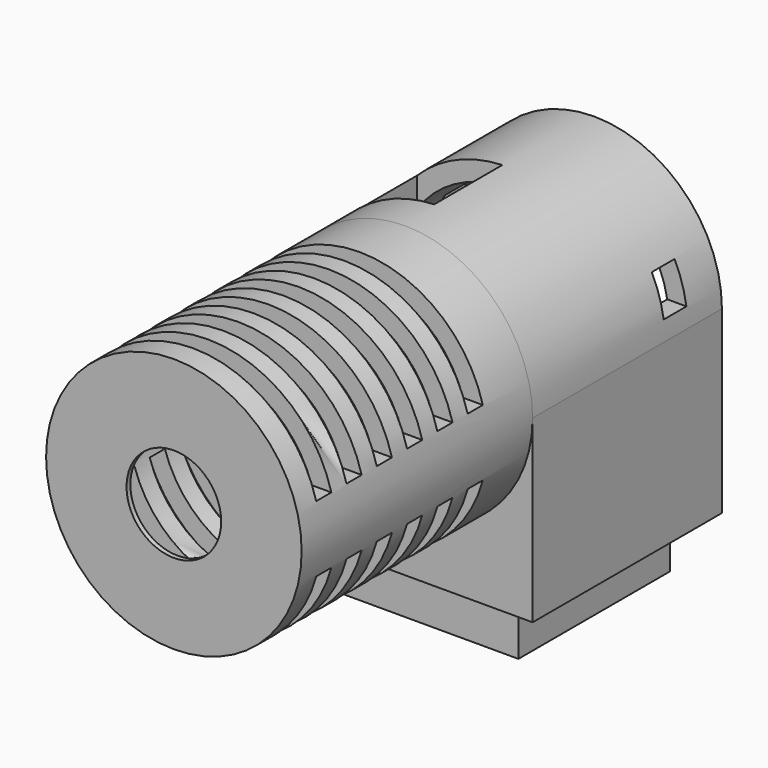
from build123d import *
from build123d import SkipClean  # not in build123d's __all__

# Parameters (mm, degrees)
F0_R      = 13.5
F0_R_2    = 11.5
F1_DEPTH  = 30
F2_R      = 13.5
F2_R_2    = 5
F3_DEPTH  = 0.5
F5_W      = 27
F5_H      = 2
F6_DEPTH  = 10
F8_W      = 27
F8_H      = 2
F9_DEPTH  = 10
F11_DEPTH = 25
F13_DEPTH = 1
F14_W     = 20
F14_H     = 20
F15_DEPTH = 5.55625
F16_W     = 3
F16_H     = 4
F17_DEPTH = 4
F18_W     = 3
F18_H     = 4
F19_DEPTH = 4
F20_W     = 9
F20_H     = 9
F21_DEPTH = 8


# Not quite as in the source:
# - after a boolean that leaves OpenCascade's solid faulty, fix() repairs it
# - a length typed as a fraction of an inch, garbled in the dataset ("3 / 203.2 mm" for 3/8 in), is restored


with BuildPart() as f1:
    # F0 (on Front) → F1 (new body)
    with BuildSketch(Plane.XZ):
        Circle(F0_R)
        Circle(F0_R_2, mode=Mode.SUBTRACT)
    extrude(amount=-F1_DEPTH)

    # F2 (on Front) → F3 (join)
    with BuildSketch(Plane.XZ):
        Circle(F2_R)
        Circle(F2_R_2, mode=Mode.SUBTRACT)
    extrude(amount=F3_DEPTH)

    # F5 (on offset) → F6 (cut)
    with BuildSketch(Plane.XY.offset(13.5)):
        with Locations((0, 2.9999998671)):
            Rectangle(F5_W, F5_H)
        with Locations((0, 22.9999998671)):
            Rectangle(F5_W, F5_H)
        with Locations((0, 6.9999998671)):
            Rectangle(F5_W, F5_H)
        with Locations((0, 10.9999998671)):
            Rectangle(F5_W, F5_H)
        with Locations((0, 14.9999998671)):
            Rectangle(F5_W, F5_H)
        with Locations((0, 18.9999998671)):
            Rectangle(F5_W, F5_H)
    extrude(amount=-F6_DEPTH, mode=Mode.SUBTRACT)

    # F8 (on offset) → F9 (cut)
    with BuildSketch(Plane.XY.offset(-13.5)):
        with Locations((5.811e-07, 3.000000095)):
            Rectangle(F8_W, F8_H)
        with Locations((5.811e-07, 7.000000095)):
            Rectangle(F8_W, F8_H)
        with Locations((5.811e-07, 11.000000095)):
            Rectangle(F8_W, F8_H)
        with Locations((5.811e-07, 15.000000095)):
            Rectangle(F8_W, F8_H)
        with Locations((5.811e-07, 19.000000095)):
            Rectangle(F8_W, F8_H)
        with Locations((5.811e-07, 23.000000095)):
            Rectangle(F8_W, F8_H)
    extrude(amount=F9_DEPTH, mode=Mode.SUBTRACT)

    # F10 (on face) → F11 (join)
    with BuildSketch(Plane(origin=(0, 30, 0), x_dir=(-1, 0, 0), z_dir=(0, 1, 0))):
        with BuildLine():
            Line((11.5, 0), (11.5, -7.0710678119))
            ThreePointArc((11.5, -7.0710678119), (12.9903810568, -3.6742346142), (13.5, 0))
            ThreePointArc((13.5, 0), (0, 13.5), (-13.5, 0))
            ThreePointArc((-13.5, 0), (-12.9903810568, -3.6742346142), (-11.5, -7.0710678119))
            Line((-11.5, -7.0710678119), (-11.5, 0))
            ThreePointArc((-11.5, 0), (0, 11.5), (11.5, 0))
        make_face()
        with BuildLine():
            ThreePointArc((13.5, 0), (12.9903810568, -3.6742346142), (11.5, -7.0710678119))
            Line((11.5, -7.0710678119), (11.5, -17))
            Line((11.5, -17), (-11.5, -17))
            Line((-11.5, -17), (-11.5, -7.0710678119))
            ThreePointArc((-11.5, -7.0710678119), (-12.9903810568, -3.6742346142), (-13.5, 0))
            Line((-13.5, 0), (-13.5, -19))
            Line((-13.5, -19), (13.5, -19))
            Line((13.5, -19), (13.5, 0))
        make_face()
    with SkipClean():  # cleaning this boolean's faces spoils the solid; the shape is the same uncleaned
        extrude(amount=F11_DEPTH)

    # F12 (on face) → F13 (join)
    with BuildSketch(Plane(origin=(0, 30, 0), x_dir=(-1, 0, 0), z_dir=(0, 1, 0))):
        with BuildLine():
            Line((13.5, -19), (13.5, 0))
            ThreePointArc((13.5, 0), (12.9903810568, -3.6742346142), (11.5, -7.0710678119))
            ThreePointArc((11.5, -7.0710678119), (0, -13.5), (-11.5, -7.0710678119))
            ThreePointArc((-11.5, -7.0710678119), (-12.9903810568, -3.6742346142), (-13.5, 0))
            Line((-13.5, 0), (-13.5, -19))
            Line((-13.5, -19), (13.5, -19))
        make_face()
        with BuildLine():
            ThreePointArc((-11.5, -7.0710678119), (0, -13.5), (11.5, -7.0710678119))
            Line((11.5, -7.0710678119), (11.5, 0))
            ThreePointArc((11.5, 0), (0, -11.5), (-11.5, 0))
            Line((-11.5, 0), (-11.5, -7.0710678119))
        make_face()
    with SkipClean():  # cleaning this boolean's faces spoils the solid; the shape is the same uncleaned
        extrude(amount=F13_DEPTH)

    # F14 (on face) → F15 (join)
    with BuildSketch(Plane(origin=(0, 0, -19), x_dir=(1, 0, 0), z_dir=(0, 0, -1))):
        with Locations((0, -42.5)):
            Rectangle(F14_W, F14_H)
        Polygon((-3.6661742094, -36.15), (3.6661742094, -36.15), (7.3323484187, -42.5), (3.6661742094, -48.85), (-3.6661742094, -48.85), (-7.3323484187, -42.5), align=None, mode=Mode.SUBTRACT)
    extrude(amount=F15_DEPTH)

    add(f1.part.fix(), mode=Mode.REPLACE)

    # F16 (on face) → F17 (cut)
    with BuildSketch(Plane.YZ.offset(13.5)):
        with Locations((49, 4)):
            Rectangle(F16_W, F16_H)
    extrude(amount=-F17_DEPTH, mode=Mode.SUBTRACT)

    # F18 (on face) → F19 (cut)
    with BuildSketch(Plane(origin=(-13.5, 0, 0), x_dir=(0, -1, 0), z_dir=(-1, 0, 0))):
        with Locations((-49, 4)):
            Rectangle(F18_W, F18_H)
    extrude(amount=-F19_DEPTH, mode=Mode.SUBTRACT)

    # F20 (on offset) → F21 (cut)
    with BuildSketch(Plane.XY.offset(13.5)):
        with Locations((-5, 39)):
            Rectangle(F20_W, F20_H)
    extrude(amount=-F21_DEPTH, mode=Mode.SUBTRACT)


solid = f1.part
